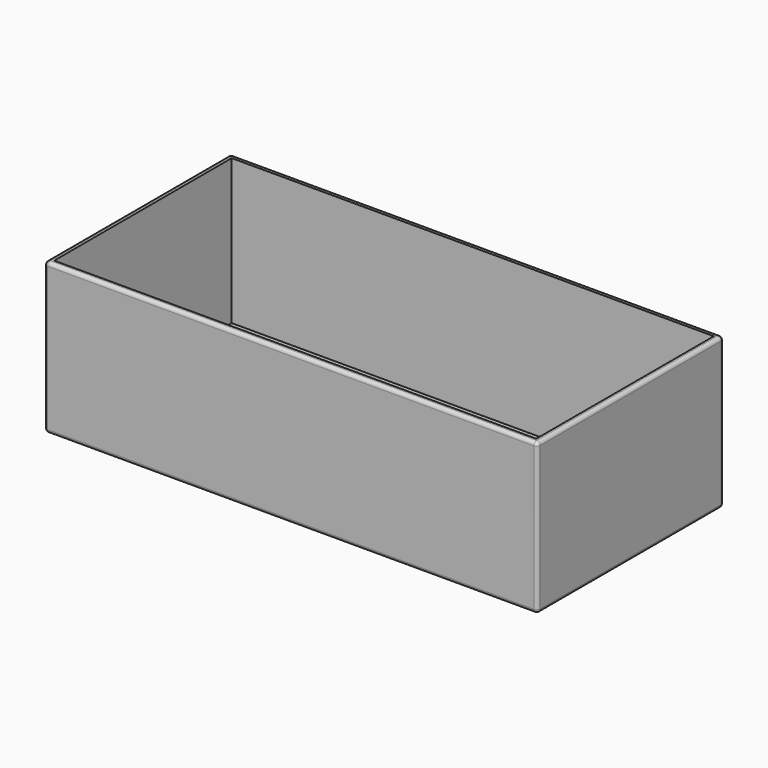
from build123d import *

# Parameters (mm, degrees)
F0_W         = 360
F0_H         = 170
F1_DEPTH     = 110
F2_T         = -4
F3_TEXT_SIZE = 31.1903241608
F4_DEPTH     = 1
F5_R         = 2.5
F6_R         = 2.5
F7_T1_DEPTH  = 105
F7_T3_DEPTH  = 355
F7_S7_W      = 2.5
F7_S7_H      = 2.5
F7_T8_DEPTH  = 2.5
F7_S13_W     = 2.5
F7_S13_H     = 2.5
F7_T14_DEPTH = 2.5
F7_S19_W     = 2.5
F7_S19_H     = 2.5
F7_T20_DEPTH = 2.5
F7_S25_W     = 2.5
F7_S25_H     = 2.5
F7_T26_DEPTH = 2.5
F7_S31_W     = 2.5
F7_S31_H     = 2.5
F7_T32_DEPTH = 2.5
F7_S37_W     = 2.5
F7_S37_H     = 2.5
F7_T38_DEPTH = 2.5
F7_T42_ANGLE = 90
F7_T44_ANGLE = 90


# Not quite as in the source:
# - a fillet or chamfer that OpenCascade refuses, or shapes differently, is made with other operations: its cross-section is extruded or revolved along the edge and cut away or added
# - Text() gives the source's letters only with a copy of the font that has no kerning and outlines rounded to 1/6400 em; it was checked with that copy


with BuildPart() as f1:
    # F0 (on Top) → F1 (new body)
    with BuildSketch(Plane.XY):
        with Locations((126.0364170372, -60.2135779709)):
            Rectangle(F0_W, F0_H)
    extrude(amount=F1_DEPTH)

    # F2
    f2_openings = [f1.faces().sort_by_distance(p)[0] for p in [
        (126.036417, -60.213578, 110),
    ]]
    offset(amount=F2_T, openings=f2_openings)

    # F3 (on face) → F4 (cut)
    with BuildSketch(Plane(origin=(0, 0, 0), x_dir=(1, 0, 0), z_dir=(0, 0, -1))):
        with Locations((61.3122358918, 62.1657297015)):
            Text('Kogi Ison', F3_TEXT_SIZE, font='Open Sans', text_align=(TextAlign.LEFT, TextAlign.BOTTOM))
    extrude(amount=-F4_DEPTH, mode=Mode.SUBTRACT)

    # F5
    f5_edges = [f1.edges().sort_by_distance(p)[0] for p in [
        (126.036417, 24.786422, 110),
        (-53.963583, -60.213578, 110),
        (306.036417, -60.213578, 110),
        (126.036417, -145.213578, 110),
    ]]
    fillet(f5_edges, radius=F5_R)

    # F6
    f6_edges = [f1.edges().sort_by_distance(p)[0] for p in [
        (-53.963583, -60.213578, 0),
        (126.036417, 24.786422, 0),
        (306.036417, -60.213578, 0),
    ]]
    fillet(f6_edges, radius=F6_R)

    # F7: fillet of radius 2.5 on 4 edges, made by hand

    # F7_s2 → F7_t1 (cut)
    with BuildSketch(Plane.XY.offset(2.5)):
        with BuildLine():
            ThreePointArc((303.5364170372, 24.7864220291), (305.3041839902, 24.0541889821), (306.0364170372, 22.2864220291))
            Line((306.0364170372, 22.2864220291), (306.0364170372, 24.7864220291))
            Line((306.0364170372, 24.7864220291), (303.5364170372, 24.7864220291))
        make_face()
        with BuildLine():
            ThreePointArc((-51.4635829628, 24.7864220291), (-53.2313499157, 24.0541889821), (-53.9635829628, 22.2864220291))
            Line((-53.9635829628, 22.2864220291), (-53.9635829628, 24.7864220291))
            Line((-53.9635829628, 24.7864220291), (-51.4635829628, 24.7864220291))
        make_face()
        with BuildLine():
            ThreePointArc((-53.9635829628, -142.7135779709), (-53.2313499157, -144.4813449238), (-51.4635829628, -145.2135779709))
            Line((-51.4635829628, -145.2135779709), (-53.9635829628, -145.2135779709))
            Line((-53.9635829628, -145.2135779709), (-53.9635829628, -142.7135779709))
        make_face()
        with BuildLine():
            ThreePointArc((306.0364170372, -142.7135779709), (305.3041839902, -144.4813449238), (303.5364170372, -145.2135779709))
            Line((303.5364170372, -145.2135779709), (306.0364170372, -145.2135779709))
            Line((306.0364170372, -145.2135779709), (306.0364170372, -142.7135779709))
        make_face()
    extrude(amount=F7_T1_DEPTH, mode=Mode.SUBTRACT)

    # F7_s4 → F7_t3 (cut)
    with BuildSketch(Plane.YZ.offset(-51.4635829628)):
        with BuildLine():
            ThreePointArc((-145.2135779709, 2.5), (-144.4813449238, 0.732233047), (-142.7135779709, 0))
            Line((-142.7135779709, 0), (-145.2135779709, 0))
            Line((-145.2135779709, 0), (-145.2135779709, 2.5))
        make_face()
    extrude(amount=F7_T3_DEPTH, mode=Mode.SUBTRACT)


with BuildPart() as f7_tool6:
    # F7_s7 → F7_t8 (new body)
    with BuildSketch(Plane.YZ.offset(303.5364170372)):
        with Locations((-143.9635779709, 108.75)):
            Rectangle(F7_S7_W, F7_S7_H)
    extrude(amount=F7_T8_DEPTH)

    # F7_s9 → F7_t10 (revolve, cut)
    with BuildSketch(Plane(origin=(303.5364170372, -142.7135779709, 107.5), x_dir=(0, 0.7071067812, -0.7071067812), z_dir=(0, -0.7071067812, -0.7071067812))):
        with BuildLine():
            ThreePointArc((0, -2.5), (2.5, 0), (0, 2.5))
            Line((0, 2.5), (0, -2.5))
        make_face()
    revolve(axis=Axis((303.5364170372, -142.7135779709, 107.5), (1, 0, 0)), mode=Mode.SUBTRACT)


with BuildPart() as f1_1:
    add(f1.part)

    # F7_t5: cut F7_tool6
    add(f7_tool6.part, mode=Mode.SUBTRACT)


with BuildPart() as f7_tool12:
    # F7_s13 → F7_t14 (new body)
    with BuildSketch(Plane.YZ.offset(-51.4635829628)):
        with Locations((-143.9635779709, 108.75)):
            Rectangle(F7_S13_W, F7_S13_H)
    extrude(amount=-F7_T14_DEPTH)

    # F7_s15 → F7_t16 (revolve, cut)
    with BuildSketch(Plane(origin=(-51.4635829628, -142.7135779709, 107.5), x_dir=(0, 0.7071067812, -0.7071067812), z_dir=(0, 0.7071067812, 0.7071067812))):
        with BuildLine():
            ThreePointArc((0, -2.5), (2.5, 0), (0, 2.5))
            Line((0, 2.5), (0, -2.5))
        make_face()
    revolve(axis=Axis((-51.4635829628, -142.7135779709, 107.5), (-1, 0, 0)), mode=Mode.SUBTRACT)


with BuildPart() as f1_2:
    add(f1_1.part)

    # F7_t11: cut F7_tool12
    add(f7_tool12.part, mode=Mode.SUBTRACT)


with BuildPart() as f7_tool18:
    # F7_s19 → F7_t20 (new body)
    with BuildSketch(Plane.XZ.offset(-22.2864220291)):
        with Locations((-52.7135829628, 1.25)):
            Rectangle(F7_S19_W, F7_S19_H)
    extrude(amount=-F7_T20_DEPTH)

    # F7_s21 → F7_t22 (revolve, cut)
    with BuildSketch(Plane(origin=(-51.4635829628, 22.2864220291, 2.5), x_dir=(0.7071067812, 0, 0.7071067812), z_dir=(-0.7071067812, 0, 0.7071067812))):
        with BuildLine():
            ThreePointArc((0, -2.5), (2.5, 0), (0, 2.5))
            Line((0, 2.5), (0, -2.5))
        make_face()
    revolve(axis=Axis((-51.4635829628, 22.2864220291, 2.5), (0, 1, 0)), mode=Mode.SUBTRACT)


with BuildPart() as f1_3:
    add(f1_2.part)

    # F7_t17: cut F7_tool18
    add(f7_tool18.part, mode=Mode.SUBTRACT)


with BuildPart() as f7_tool24:
    # F7_s25 → F7_t26 (new body)
    with BuildSketch(Plane.XZ.offset(-22.2864220291)):
        with Locations((-52.7135829628, 108.75)):
            Rectangle(F7_S25_W, F7_S25_H)
    extrude(amount=-F7_T26_DEPTH)

    # F7_s27 → F7_t28 (revolve, cut)
    with BuildSketch(Plane(origin=(-51.4635829628, 22.2864220291, 107.5), x_dir=(0.7071067812, 0, -0.7071067812), z_dir=(0.7071067812, 0, 0.7071067812))):
        with BuildLine():
            ThreePointArc((0, -2.5), (2.5, 0), (0, 2.5))
            Line((0, 2.5), (0, -2.5))
        make_face()
    revolve(axis=Axis((-51.4635829628, 22.2864220291, 107.5), (0, 1, 0)), mode=Mode.SUBTRACT)


with BuildPart() as f1_4:
    add(f1_3.part)

    # F7_t23: cut F7_tool24
    add(f7_tool24.part, mode=Mode.SUBTRACT)


with BuildPart() as f7_tool30:
    # F7_s31 → F7_t32 (new body)
    with BuildSketch(Plane.XZ.offset(-22.2864220291)):
        with Locations((304.7864170372, 1.25)):
            Rectangle(F7_S31_W, F7_S31_H)
    extrude(amount=-F7_T32_DEPTH)

    # F7_s33 → F7_t34 (revolve, cut)
    with BuildSketch(Plane(origin=(303.5364170372, 22.2864220291, 2.5), x_dir=(-0.7071067812, 0, 0.7071067812), z_dir=(-0.7071067812, 0, -0.7071067812))):
        with BuildLine():
            ThreePointArc((0, -2.5), (2.5, 0), (0, 2.5))
            Line((0, 2.5), (0, -2.5))
        make_face()
    revolve(axis=Axis((303.5364170372, 22.2864220291, 2.5), (0, 1, 0)), mode=Mode.SUBTRACT)


with BuildPart() as f1_5:
    add(f1_4.part)

    # F7_t29: cut F7_tool30
    add(f7_tool30.part, mode=Mode.SUBTRACT)


with BuildPart() as f7_tool36:
    # F7_s37 → F7_t38 (new body)
    with BuildSketch(Plane.XZ.offset(-22.2864220291)):
        with Locations((304.7864170372, 108.75)):
            Rectangle(F7_S37_W, F7_S37_H)
    extrude(amount=-F7_T38_DEPTH)

    # F7_s39 → F7_t40 (revolve, cut)
    with BuildSketch(Plane(origin=(303.5364170372, 22.2864220291, 107.5), x_dir=(-0.7071067812, 0, -0.7071067812), z_dir=(0.7071067812, 0, -0.7071067812))):
        with BuildLine():
            ThreePointArc((0, -2.5), (2.5, 0), (0, 2.5))
            Line((0, 2.5), (0, -2.5))
        make_face()
    revolve(axis=Axis((303.5364170372, 22.2864220291, 107.5), (0, 1, 0)), mode=Mode.SUBTRACT)


with BuildPart() as f1_6:
    add(f1_5.part)

    # F7_t35: cut F7_tool36
    add(f7_tool36.part, mode=Mode.SUBTRACT)

    # F7_s41 → F7_t42 (revolve, cut)
    with BuildSketch(Plane.XY.offset(2.5)):
        with BuildLine():
            ThreePointArc((303.5364170372, -145.2135779709), (305.3041839902, -144.4813449238), (306.0364170372, -142.7135779709))
            Line((306.0364170372, -142.7135779709), (306.0364170372, -145.2135779709))
            Line((306.0364170372, -145.2135779709), (303.5364170372, -145.2135779709))
        make_face()
    revolve(axis=Axis((303.5364170372, -145.2135779709, 2.5), (0, 1, 0)), revolution_arc=F7_T42_ANGLE, mode=Mode.SUBTRACT)

    # F7_s43 → F7_t44 (revolve, cut)
    with BuildSketch(Plane.YZ.offset(-51.4635829628)):
        with BuildLine():
            ThreePointArc((-145.2135779709, 2.5), (-144.4813449238, 0.732233047), (-142.7135779709, 0))
            Line((-142.7135779709, 0), (-145.2135779709, 0))
            Line((-145.2135779709, 0), (-145.2135779709, 2.5))
        make_face()
    revolve(axis=Axis((-51.4635829628, -145.2135779709, 2.5), (0, 1, 0)), revolution_arc=F7_T44_ANGLE, mode=Mode.SUBTRACT)


solid = f1_6.part
